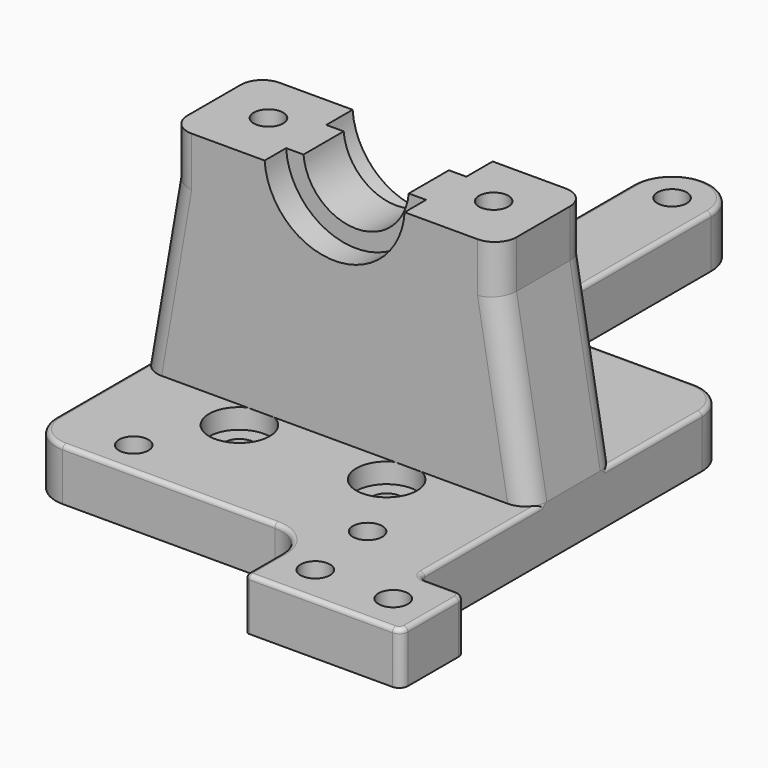
from build123d import *

# Parameters (mm, degrees)
F1_R           = 1.7
F2_DEPTH       = 6
F4_D           = 3.4
F4_CBORE_D     = 7
F4_CBORE_DEPTH = 2.3
F7_DEPTH       = 12.7
F8_R           = 2.5
F9_T1_DEPTH    = 24.5
F9_T3_DEPTH    = 12.12
F9_T5_DEPTH    = 12.18
F9_T7_DEPTH    = 27
F9_T9_DEPTH    = 4.8
F9_T11_DEPTH   = 16.5
F9_T13_DEPTH   = 15.12
F9_T15_DEPTH   = 7.3
F9_T17_DEPTH   = 3.5
F9_T19_DEPTH   = 19.75
F9_T21_DEPTH   = 8.25
F9_T26_DEPTH   = 2.5
F9_S27_R       = 2.5
F9_T28_DEPTH   = 3
F9_T32_DEPTH   = 2.5
F9_S33_R       = 2.5
F9_T34_DEPTH   = 3
F9_T36_ANGLE   = 90
F9_T40_DEPTH   = 2.5
F9_S41_R       = 2.5
F9_T42_DEPTH   = 3
F9_T46_DEPTH   = 2.5
F9_S47_R       = 2.5
F9_T48_DEPTH   = 3
F9_T50_ANGLE   = 90
F9_T52_ANGLE   = 90
F9_T54_ANGLE   = 90
F9_T56_ANGLE   = 90
F9_T58_ANGLE   = 90
F9_T60_ANGLE   = 90
F9_T62_ANGLE   = 180
F9_T64_ANGLE   = 90
F9_T69_DEPTH   = 28.25
F9_T73_DEPTH   = 9.5
F9_T80_DEPTH   = 21
F9_T84_DEPTH   = 28.25
F11_D          = 3.4
F11_DEPTH      = 12
F11_TIP        = 1.0214630523
F13_DEPTH      = 3.1
F15_DEPTH      = 3.8


# Not quite as in the source:
# - a fillet or chamfer that OpenCascade refuses, or shapes differently, is made with other operations: its cross-section is extruded or revolved along the edge and cut away or added
# - a feature names something its author has since deleted; it is built from what else it names


with BuildPart() as f2:
    # F1 (on offset) → F2 (new body)
    with BuildSketch(Plane.XY.offset(-16)):
        with BuildLine():
            Line((-22.5, 7.38), (-22.5, -29.62))
            ThreePointArc((-22.5, -29.62), (-21.3284271247, -32.4484271247), (-18.5, -33.62))
            Line((-18.5, -33.62), (6, -33.62))
            ThreePointArc((6, -33.62), (8.8284271247, -34.7915728753), (10, -37.62))
            Line((10, -37.62), (10, -42.42))
            ThreePointArc((10, -42.42), (10.1464466094, -42.7735533906), (10.5, -42.92))
            Line((10.5, -42.92), (17.4366980791, -42.92))
            Line((17.4366980791, -42.92), (22, -42.92))
            Line((22, -42.92), (27, -42.92))
            ThreePointArc((27, -42.92), (27.7071067812, -42.6271067812), (28, -41.92))
            Line((28, -41.92), (28, -34.62))
            ThreePointArc((28, -34.62), (27.7071067812, -33.9128932188), (27, -33.62))
            Line((27, -33.62), (23.5, -33.62))
            ThreePointArc((23.5, -33.62), (22.7928932188, -33.3271067812), (22.5, -32.62))
            Line((22.5, -32.62), (22.5, 7.38))
            ThreePointArc((22.5, 7.38), (21.3284271247, 10.2084271247), (18.5, 11.38))
            Line((18.5, 11.38), (-1.25, 11.38))
            Line((-1.25, 11.38), (-10.25, 11.38))
            Line((-10.25, 11.38), (-18.5, 11.38))
            ThreePointArc((-18.5, 11.38), (-21.3284271247, 10.2084271247), (-22.5, 7.38))
        make_face()
        with Locations((-13.5, -29.62)):
            Circle(F1_R, mode=Mode.SUBTRACT)
        with Locations((-8.5, -20.62)):
            Circle(F1_R, mode=Mode.SUBTRACT)
        with Locations((-8.5, -1.62)):
            Circle(F1_R, mode=Mode.SUBTRACT)
        with Locations((14.5, -38.42)):
            Circle(F1_R, mode=Mode.SUBTRACT)
        with Locations((13.5, -29.62)):
            Circle(F1_R, mode=Mode.SUBTRACT)
        with Locations((23.5, -38.42)):
            Circle(F1_R, mode=Mode.SUBTRACT)
        with Locations((8.5, -20.62)):
            Circle(F1_R, mode=Mode.SUBTRACT)
        with Locations((8.5, -1.62)):
            Circle(F1_R, mode=Mode.SUBTRACT)
        with BuildLine():
            Line((-10.25, 38.38), (-10.25, 11.38))
            Line((-10.25, 11.38), (-1.25, 11.38))
            Line((-1.25, 11.38), (-1.25, 38.38))
            ThreePointArc((-1.25, 38.38), (-5.75, 42.88), (-10.25, 38.38))
        make_face()
        with Locations((-5.75, 38.38)):
            Circle(F1_R, mode=Mode.SUBTRACT)
    extrude(amount=F2_DEPTH)

    # F4 (through all)
    with Locations(Plane.XY.offset(-10)):
        with Locations((-8.5, -1.62), (8.5, -1.62), (-8.5, -20.62), (8.5, -20.62)):
            CounterBoreHole(F4_D / 2, F4_CBORE_D / 2, F4_CBORE_DEPTH)

    # F6 (on offset) → F7 (join)
    with BuildSketch(Plane.XZ.offset(4.8)):
        with BuildLine():
            Line((9.75, -10), (22.5, -10))
            Line((22.5, -10), (19, 10.25))
            Line((19, 10.25), (19, 15.75))
            Line((19, 15.75), (6.0762101901, 15.75))
            ThreePointArc((6.0762101901, 15.75), (0, 10.1882097417), (-6.0762101901, 15.75))
            Line((-6.0762101901, 15.75), (-19, 15.75))
            Line((-19, 15.75), (-19, 10.25))
            Line((-19, 10.25), (-22.5, -10))
            Line((-22.5, -10), (-9.75, -10))
            Line((-9.75, -10), (9.75, -10))
        make_face()
    extrude(amount=F7_DEPTH)

    # F8
    f8_edges = [f2.edges().sort_by_distance(p)[0] for p in [
        (20.75, -17.5, 0.125),
        (19, -17.5, 13),
        (20.75, -4.8, 0.125),
        (19, -4.8, 13),
        (-20.75, -4.8, 0.125),
        (-19, -4.8, 13),
        (-20.75, -17.5, 0.125),
        (-19, -17.5, 13),
    ]]
    fillet(f8_edges, radius=F8_R)

    # F9: fillet of radius 0.5 on 26 edges, made by hand

    # F9_s2 → F9_t1 (cut)
    with BuildSketch(Plane.YZ.offset(-18.5)):
        with BuildLine():
            ThreePointArc((-33.12, -10), (-33.4735533906, -10.1464466094), (-33.62, -10.5))
            Line((-33.62, -10.5), (-33.62, -10))
            Line((-33.62, -10), (-33.12, -10))
        make_face()
    extrude(amount=F9_T1_DEPTH, mode=Mode.SUBTRACT)

    # F9_s4 → F9_t3 (cut)
    with BuildSketch(Plane.XZ.offset(17.5)):
        with BuildLine():
            ThreePointArc((-22, -10), (-22.3535533906, -10.1464466094), (-22.5, -10.5))
            Line((-22.5, -10.5), (-22.5, -10))
            Line((-22.5, -10), (-22, -10))
        make_face()
    extrude(amount=F9_T3_DEPTH, mode=Mode.SUBTRACT)

    # F9_s6 → F9_t5 (cut)
    with BuildSketch(Plane.XZ.offset(-7.38)):
        with BuildLine():
            ThreePointArc((-22.5, -10.5), (-22.3535533906, -10.1464466094), (-22, -10))
            Line((-22, -10), (-22.5, -10))
            Line((-22.5, -10), (-22.5, -10.5))
        make_face()
        with BuildLine():
            ThreePointArc((22.5, -10.5), (22.3535533906, -10.1464466094), (22, -10))
            Line((22, -10), (22.5, -10))
            Line((22.5, -10), (22.5, -10.5))
        make_face()
    extrude(amount=F9_T5_DEPTH, mode=Mode.SUBTRACT)

    # F9_s8 → F9_t7 (cut)
    with BuildSketch(Plane.XZ.offset(-38.38)):
        with BuildLine():
            ThreePointArc((-9.75, -10), (-10.1035533906, -10.1464466094), (-10.25, -10.5))
            Line((-10.25, -10.5), (-10.25, -10))
            Line((-10.25, -10), (-9.75, -10))
        make_face()
        with BuildLine():
            ThreePointArc((-1.75, -10), (-1.3964466094, -10.1464466094), (-1.25, -10.5))
            Line((-1.25, -10.5), (-1.25, -10))
            Line((-1.25, -10), (-1.75, -10))
        make_face()
    extrude(amount=F9_T7_DEPTH, mode=Mode.SUBTRACT)

    # F9_s10 → F9_t9 (cut)
    with BuildSketch(Plane.XZ.offset(37.62)):
        with BuildLine():
            ThreePointArc((10.5, -10), (10.1464466094, -10.1464466094), (10, -10.5))
            Line((10, -10.5), (10, -10))
            Line((10, -10), (10.5, -10))
        make_face()
    extrude(amount=F9_T9_DEPTH, mode=Mode.SUBTRACT)

    # F9_s12 → F9_t11 (cut)
    with BuildSketch(Plane.YZ.offset(10.5)):
        with BuildLine():
            ThreePointArc((-42.42, -10), (-42.7735533906, -10.1464466094), (-42.92, -10.5))
            Line((-42.92, -10.5), (-42.92, -10))
            Line((-42.92, -10), (-42.42, -10))
        make_face()
    extrude(amount=F9_T11_DEPTH, mode=Mode.SUBTRACT)

    # F9_s14 → F9_t13 (cut)
    with BuildSketch(Plane.XZ.offset(17.5)):
        with BuildLine():
            ThreePointArc((22, -10), (22.3535533906, -10.1464466094), (22.5, -10.5))
            Line((22.5, -10.5), (22.5, -10))
            Line((22.5, -10), (22, -10))
        make_face()
    extrude(amount=F9_T13_DEPTH, mode=Mode.SUBTRACT)

    # F9_s16 → F9_t15 (cut)
    with BuildSketch(Plane.XZ.offset(34.62)):
        with BuildLine():
            ThreePointArc((27.5, -10), (27.8535533906, -10.1464466094), (28, -10.5))
            Line((28, -10.5), (28, -10))
            Line((28, -10), (27.5, -10))
        make_face()
    extrude(amount=F9_T15_DEPTH, mode=Mode.SUBTRACT)

    # F9_s18 → F9_t17 (cut)
    with BuildSketch(Plane.YZ.offset(23.5)):
        with BuildLine():
            ThreePointArc((-34.12, -10), (-33.7664466094, -10.1464466094), (-33.62, -10.5))
            Line((-33.62, -10.5), (-33.62, -10))
            Line((-33.62, -10), (-34.12, -10))
        make_face()
    extrude(amount=F9_T17_DEPTH, mode=Mode.SUBTRACT)

    # F9_s20 → F9_t19 (cut)
    with BuildSketch(Plane.YZ.offset(-1.25)):
        with BuildLine():
            ThreePointArc((10.88, -10), (11.2335533906, -10.1464466094), (11.38, -10.5))
            Line((11.38, -10.5), (11.38, -10))
            Line((11.38, -10), (10.88, -10))
        make_face()
    extrude(amount=F9_T19_DEPTH, mode=Mode.SUBTRACT)

    # F9_s22 → F9_t21 (cut)
    with BuildSketch(Plane.YZ.offset(-18.5)):
        with BuildLine():
            ThreePointArc((10.88, -10), (11.2335533906, -10.1464466094), (11.38, -10.5))
            Line((11.38, -10.5), (11.38, -10))
            Line((11.38, -10), (10.88, -10))
        make_face()
    extrude(amount=F9_T21_DEPTH, mode=Mode.SUBTRACT)


with BuildPart() as f9_tool24:
    # F9_s25 → F9_t26 (new body)
    with BuildSketch(Plane.XZ.offset(17.5)):
        with BuildLine():
            ThreePointArc((22, -10), (22.3535533906, -10.1464466094), (22.5, -10.5))
            Line((22.5, -10.5), (22.5, -10))
            Line((22.5, -10), (22, -10))
        make_face()
    extrude(amount=-F9_T26_DEPTH)

    # F9_s27 → F9_t28 (cut, symmetric)
    with BuildSketch(Plane(origin=(2.3673685645, 0, -13.6969181234), x_dir=(0, 1, 0), z_dir=(-0.1703142852, 0, 0.9853897931))):
        with Locations((-15, -17.9681274915)):
            Circle(F9_S27_R)
    extrude(amount=F9_T28_DEPTH, both=True, mode=Mode.SUBTRACT)


with BuildPart() as f2_1:
    add(f2.part)

    # F9_t23: cut F9_tool24
    add(f9_tool24.part, mode=Mode.SUBTRACT)


with BuildPart() as f9_tool30:
    # F9_s31 → F9_t32 (new body)
    with BuildSketch(Plane.XZ.offset(7.3)):
        with BuildLine():
            ThreePointArc((22.5, -10.5), (22.3535533906, -10.1464466094), (22, -10))
            Line((22, -10), (22.5, -10))
            Line((22.5, -10), (22.5, -10.5))
        make_face()
    extrude(amount=-F9_T32_DEPTH)

    # F9_s33 → F9_t34 (cut, symmetric)
    with BuildSketch(Plane(origin=(2.3673685645, 0, -13.6969181234), x_dir=(0, 1, 0), z_dir=(-0.1703142852, 0, 0.9853897931))):
        with Locations((-7.3, -17.9681274915)):
            Circle(F9_S33_R)
    extrude(amount=F9_T34_DEPTH, both=True, mode=Mode.SUBTRACT)


with BuildPart() as f2_2:
    add(f2_1.part)

    # F9_t29: cut F9_tool30
    add(f9_tool30.part, mode=Mode.SUBTRACT)

    # F9_s35 → F9_t36 (revolve, cut)
    with BuildSketch(Plane.XZ.offset(29.62)):
        with BuildLine():
            ThreePointArc((-22, -10), (-22.3535533906, -10.1464466094), (-22.5, -10.5))
            Line((-22.5, -10.5), (-22.5, -10))
            Line((-22.5, -10), (-22, -10))
        make_face()
    revolve(axis=Axis((-18.5, -29.62, -10), (0, 0, 1)), revolution_arc=F9_T36_ANGLE, mode=Mode.SUBTRACT)


with BuildPart() as f9_tool38:
    # F9_s39 → F9_t40 (new body)
    with BuildSketch(Plane.XZ.offset(15)):
        with BuildLine():
            ThreePointArc((-22, -10), (-22.3535533906, -10.1464466094), (-22.5, -10.5))
            Line((-22.5, -10.5), (-22.5, -10))
            Line((-22.5, -10), (-22, -10))
        make_face()
    extrude(amount=F9_T40_DEPTH)

    # F9_s41 → F9_t42 (cut, symmetric)
    with BuildSketch(Plane(origin=(-2.3673685645, 0, -13.6969181234), x_dir=(0, 1, 0), z_dir=(-0.1703142852, 0, -0.9853897931))):
        with Locations((-15, -17.9681274915)):
            Circle(F9_S41_R)
    extrude(amount=F9_T42_DEPTH, both=True, mode=Mode.SUBTRACT)


with BuildPart() as f2_3:
    add(f2_2.part)

    # F9_t37: cut F9_tool38
    add(f9_tool38.part, mode=Mode.SUBTRACT)


with BuildPart() as f9_tool44:
    # F9_s45 → F9_t46 (new body)
    with BuildSketch(Plane.XZ.offset(4.8)):
        with BuildLine():
            ThreePointArc((-22.5, -10.5), (-22.3535533906, -10.1464466094), (-22, -10))
            Line((-22, -10), (-22.5, -10))
            Line((-22.5, -10), (-22.5, -10.5))
        make_face()
    extrude(amount=F9_T46_DEPTH)

    # F9_s47 → F9_t48 (cut, symmetric)
    with BuildSketch(Plane(origin=(-2.3673685645, 0, -13.6969181234), x_dir=(0, 1, 0), z_dir=(-0.1703142852, 0, -0.9853897931))):
        with Locations((-7.3, -17.9681274915)):
            Circle(F9_S47_R)
    extrude(amount=F9_T48_DEPTH, both=True, mode=Mode.SUBTRACT)


with BuildPart() as f2_4:
    add(f2_3.part)

    # F9_t43: cut F9_tool44
    add(f9_tool44.part, mode=Mode.SUBTRACT)

    # F9_s49 → F9_t50 (revolve, cut)
    with BuildSketch(Plane.YZ.offset(6)):
        with BuildLine():
            ThreePointArc((-33.12, -10), (-33.4735533906, -10.1464466094), (-33.62, -10.5))
            Line((-33.62, -10.5), (-33.62, -10))
            Line((-33.62, -10), (-33.12, -10))
        make_face()
    revolve(axis=Axis((6, -37.62, -10), (0, 0, -1)), revolution_arc=F9_T50_ANGLE, mode=Mode.SUBTRACT)

    # F9_s51 → F9_t52 (revolve, cut)
    with BuildSketch(Plane.XZ.offset(42.42)):
        with BuildLine():
            ThreePointArc((10.5, -10), (10.1464466094, -10.1464466094), (10, -10.5))
            Line((10, -10.5), (10, -10))
            Line((10, -10), (10.5, -10))
        make_face()
    revolve(axis=Axis((10.5, -42.42, -10), (0, 0, 1)), revolution_arc=F9_T52_ANGLE, mode=Mode.SUBTRACT)

    # F9_s53 → F9_t54 (revolve, cut)
    with BuildSketch(Plane.YZ.offset(27)):
        with BuildLine():
            ThreePointArc((-42.42, -10), (-42.7735533906, -10.1464466094), (-42.92, -10.5))
            Line((-42.92, -10.5), (-42.92, -10))
            Line((-42.92, -10), (-42.42, -10))
        make_face()
    revolve(axis=Axis((27, -41.92, -10), (0, 0, 1)), revolution_arc=F9_T54_ANGLE, mode=Mode.SUBTRACT)

    # F9_s55 → F9_t56 (revolve, cut)
    with BuildSketch(Plane.YZ.offset(23.5)):
        with BuildLine():
            ThreePointArc((-34.12, -10), (-33.7664466094, -10.1464466094), (-33.62, -10.5))
            Line((-33.62, -10.5), (-33.62, -10))
            Line((-33.62, -10), (-34.12, -10))
        make_face()
    revolve(axis=Axis((23.5, -32.62, -10), (0, 0, -1)), revolution_arc=F9_T56_ANGLE, mode=Mode.SUBTRACT)

    # F9_s57 → F9_t58 (revolve, cut)
    with BuildSketch(Plane.XZ.offset(34.62)):
        with BuildLine():
            ThreePointArc((27.5, -10), (27.8535533906, -10.1464466094), (28, -10.5))
            Line((28, -10.5), (28, -10))
            Line((28, -10), (27.5, -10))
        make_face()
    revolve(axis=Axis((27, -34.62, -10), (0, 0, 1)), revolution_arc=F9_T58_ANGLE, mode=Mode.SUBTRACT)

    # F9_s59 → F9_t60 (revolve, cut)
    with BuildSketch(Plane.XZ.offset(-7.38)):
        with BuildLine():
            ThreePointArc((22, -10), (22.3535533906, -10.1464466094), (22.5, -10.5))
            Line((22.5, -10.5), (22.5, -10))
            Line((22.5, -10), (22, -10))
        make_face()
    revolve(axis=Axis((18.5, 7.38, -10), (0, 0, 1)), revolution_arc=F9_T60_ANGLE, mode=Mode.SUBTRACT)

    # F9_s61 → F9_t62 (revolve, cut)
    with BuildSketch(Plane.XZ.offset(-38.38)):
        with BuildLine():
            ThreePointArc((-1.75, -10), (-1.3964466094, -10.1464466094), (-1.25, -10.5))
            Line((-1.25, -10.5), (-1.25, -10))
            Line((-1.25, -10), (-1.75, -10))
        make_face()
    revolve(axis=Axis((-5.75, 38.38, -10), (0, 0, 1)), revolution_arc=F9_T62_ANGLE, mode=Mode.SUBTRACT)

    # F9_s63 → F9_t64 (revolve, cut)
    with BuildSketch(Plane.YZ.offset(-18.5)):
        with BuildLine():
            ThreePointArc((10.88, -10), (11.2335533906, -10.1464466094), (11.38, -10.5))
            Line((11.38, -10.5), (11.38, -10))
            Line((11.38, -10), (10.88, -10))
        make_face()
    revolve(axis=Axis((-18.5, 7.38, -10), (0, 0, 1)), revolution_arc=F9_T64_ANGLE, mode=Mode.SUBTRACT)


with BuildPart() as f9_tool67:
    # F9_s68 → F9_t69 (new body)
    with BuildSketch(Plane.XZ.offset(-38.38)):
        with BuildLine():
            ThreePointArc((-9.75, -10), (-10.1035533906, -10.1464466094), (-10.25, -10.5))
            Line((-10.25, -10.5), (-10.25, -10))
            Line((-10.25, -10), (-9.75, -10))
        make_face()
    extrude(amount=F9_T69_DEPTH)

    split(bisect_by=Plane.XZ.offset(-11.38), keep=Keep.TOP)


with BuildPart() as f9_tool71:
    # F9_s72 → F9_t73 (new body)
    with BuildSketch(Plane.YZ.offset(-9)):
        with BuildLine():
            ThreePointArc((10.88, -10), (11.2335533906, -10.1464466094), (11.38, -10.5))
            Line((11.38, -10.5), (11.38, -10))
            Line((11.38, -10), (10.88, -10))
        make_face()
    extrude(amount=-F9_T73_DEPTH)

    split(bisect_by=Plane.YZ.offset(-10.25), keep=Keep.TOP)


with BuildPart() as f9_tool67_1:
    add(f9_tool67.part)

    # F9_t75: intersect F9_tool71
    add(f9_tool71.part, mode=Mode.INTERSECT)


with BuildPart() as f2_5:
    add(f2_4.part)

    # F9_t65: cut F9_tool67
    add(f9_tool67_1.part, mode=Mode.SUBTRACT)


with BuildPart() as f9_tool78:
    # F9_s79 → F9_t80 (new body)
    with BuildSketch(Plane.YZ.offset(18.5)):
        with BuildLine():
            ThreePointArc((10.88, -10), (11.2335533906, -10.1464466094), (11.38, -10.5))
            Line((11.38, -10.5), (11.38, -10))
            Line((11.38, -10), (10.88, -10))
        make_face()
    extrude(amount=-F9_T80_DEPTH)

    split(bisect_by=Plane.YZ.offset(-1.25), keep=Keep.BOTTOM)


with BuildPart() as f9_tool82:
    # F9_s83 → F9_t84 (new body)
    with BuildSketch(Plane.XZ.offset(-10.13)):
        with BuildLine():
            ThreePointArc((-1.75, -10), (-1.3964466094, -10.1464466094), (-1.25, -10.5))
            Line((-1.25, -10.5), (-1.25, -10))
            Line((-1.25, -10), (-1.75, -10))
        make_face()
    extrude(amount=-F9_T84_DEPTH)

    split(bisect_by=Plane.XZ.offset(-11.38), keep=Keep.TOP)


with BuildPart() as f9_tool78_1:
    add(f9_tool78.part)

    # F9_t86: intersect F9_tool82
    add(f9_tool82.part, mode=Mode.INTERSECT)


with BuildPart() as f2_6:
    add(f2_5.part)

    # F9_t76: cut F9_tool78
    add(f9_tool78_1.part, mode=Mode.SUBTRACT)

    # F11
    with Locations(Plane.XY.offset(15.75)):
        with Locations((-13, -10.8), (13, -10.8)):
            Hole(F11_D / 2, depth=F11_DEPTH)
            with Locations((0, 0, -(F11_DEPTH + F11_TIP / 2))):  # 118° drill point
                Cone(0, F11_D / 2, F11_TIP, mode=Mode.SUBTRACT)

    # F12 (on face) → F13 (cut)
    with BuildSketch(Plane.XZ.offset(17.5)):
        with BuildLine():
            ThreePointArc((6.0762101901, 15.75), (0, 10.1882097417), (-6.0762101901, 15.75))
            Line((-6.0762101901, 15.75), (-8.0820993729, 15.75))
            ThreePointArc((-8.0820993729, 15.75), (0, 8.1882097417), (8.0820993729, 15.75))
            Line((8.0820993729, 15.75), (6.0762101901, 15.75))
        make_face()
    extrude(amount=-F13_DEPTH, mode=Mode.SUBTRACT)

    # F14 (on face) → F15 (cut)
    with BuildSketch(Plane(origin=(0, -4.8, 0), x_dir=(-1, 0, 0), z_dir=(0, 1, 0))):
        with BuildLine():
            Line((8.0820993729, 15.75), (6.0762101901, 15.75))
            ThreePointArc((6.0762101901, 15.75), (0, 10.1882097417), (-6.0762101901, 15.75))
            Line((-6.0762101901, 15.75), (-8.0820993729, 15.75))
            ThreePointArc((-8.0820993729, 15.75), (0, 8.1882097417), (8.0820993729, 15.75))
        make_face()
    extrude(amount=-F15_DEPTH, mode=Mode.SUBTRACT)


solid = f2_6.part
